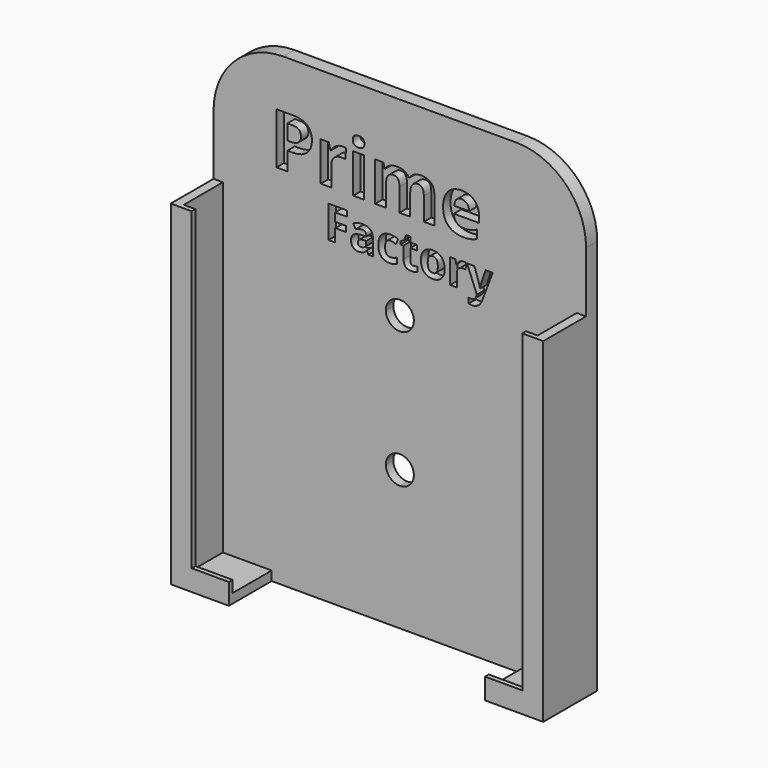
from build123d import *

# Parameters (mm, degrees)
F1_DEPTH        = 13
F3_DEPTH        = 3
F4_W            = 71
F4_H            = 4.5
F5_DEPTH        = 1
F6_R            = 15
F7_W            = 15
F7_H            = 4.5
F8_DEPTH        = 11
F10_W           = 24
F10_H           = 43
F11_DEPTH       = 1
F13_DEPTH       = 0.5
F14_DEPTH       = 30
F15_DEPTH       = 26
F16_DEPTH       = 8
F17_DEPTH       = 8
F18_TEXT_SIZE   = 15.3918698844
F18_TEXT_SIZE_2 = 9.6479482535
F19_DEPTH       = 2
F20_DEPTH       = 0.5
F21_DEPTH       = 0.5
F22_DEPTH       = 0.5
F23_DEPTH       = 0.5
F27_DEPTH       = 25
F28_DEPTH       = 25


# Not quite as in the source:
# - Text() gives the source's letters only with a copy of the font that has no kerning and outlines rounded to 1/6400 em; it was checked with that copy


with BuildPart() as f1:
    # F0 (on Front) → F1 (new body)
    with BuildSketch(Plane.XZ):
        Polygon((-38, -35), (-38, 35), (-40, 35), (-40, -37), (40, -37), (40, 35), (38, 35), (38, -35), align=None)
    extrude(amount=F1_DEPTH)

    # F2 (on face) → F3 (join)
    with BuildSketch(Plane(origin=(0, 0, 0), x_dir=(-1, 0, 0), z_dir=(0, 1, 0))):
        Polygon((-40, 63), (-40, 35), (-38, 35), (-38, -35), (38, -35), (38, 35), (40, 35), (40, 63), align=None)
    extrude(amount=-F3_DEPTH)

    # F4 (on face) → F5 (join)
    with BuildSketch(Plane.XZ.offset(13)):
        Polygon((35.5, -37), (40, -37), (40, 35), (35.5, 35), (35.5, -32.5), align=None)
        with Locations((0, -34.75)):
            Rectangle(F4_W, F4_H)
        Polygon((-40, -37), (-35.5, -37), (-35.5, -32.5), (-35.5, 35), (-40, 35), align=None)
    extrude(amount=F5_DEPTH)

    # F6
    f6_edges = [f1.edges().sort_by_distance(p)[0] for p in [
        (-40, -1.5, 63),
        (40, -1.5, 63),
    ]]
    fillet(f6_edges, radius=F6_R)

    # F7 (on face) → F8 (cut)
    with BuildSketch(Plane.XZ.offset(14)):
        with Locations((1.9808986038, -34.75)):
            Rectangle(F7_W, F7_H)
    extrude(amount=-F8_DEPTH, mode=Mode.SUBTRACT)

    # F10 (on face) → F11 (cut)
    with BuildSketch(Plane(origin=(0, 0, 0), x_dir=(-1, 0, 0), z_dir=(0, 1, 0))):
        with Locations((0, 7.5584797218)):
            Rectangle(F10_W, F10_H)
    extrude(amount=-F11_DEPTH, mode=Mode.SUBTRACT)

    # F12 (on face) → F13 (cut)
    with BuildSketch(Plane.XZ.offset(3)):
        with BuildLine():
            Line((-38, 35), (-38, -35))
            Line((-38, -35), (-5.5191013962, -35))
            Line((-5.5191013962, -35), (9.4808986038, -35))
            Line((9.4808986038, -35), (38, -35))
            Line((38, -35), (38, 35))
            Line((38, 35), (40, 35))
            Line((40, 35), (40, 48))
            ThreePointArc((40, 48), (35.6066017178, 58.6066017178), (25, 63))
            Line((25, 63), (-25, 63))
            ThreePointArc((-25, 63), (-35.6066017178, 58.6066017178), (-40, 48))
            Line((-40, 48), (-40, 35))
            Line((-40, 35), (-38, 35))
        make_face()
    extrude(amount=F13_DEPTH, mode=Mode.SUBTRACT)

    # F14 (cut): a face of the model
    f14_faces = [f1.faces().sort_by_distance(p)[0] for p in [
        (-5.5191013962, -9.0102040816, -35.7704081633),
    ]]
    extrude(f14_faces, amount=-F14_DEPTH, mode=Mode.SUBTRACT)

    # F15 (cut): a face of the model
    f15_faces = [f1.faces().sort_by_distance(p)[0] for p in [
        (9.4808986038, -9.0102040816, -35.7704081633),
    ]]
    extrude(f15_faces, amount=-F15_DEPTH, mode=Mode.SUBTRACT)

    # F16 (add): a face of the model
    f16_faces = [f1.faces().sort_by_distance(p)[0] for p in [
        (35.4808986038, -9.0102040816, -35.7704081633),
    ]]
    extrude(f16_faces, amount=F16_DEPTH)

    # F17 (add): a face of the model
    f17_faces = [f1.faces().sort_by_distance(p)[0] for p in [
        (-35.5191013962, -9.0102040816, -35.7704081633),
    ]]
    extrude(f17_faces, amount=F17_DEPTH)

    # F18 (on face) → F19 (cut)
    with BuildSketch(Plane.XZ.offset(3)):
        with Locations((-27.8627396328, 41.5634587407)):
            Text('Prime', F18_TEXT_SIZE, font='Open Sans', font_style=FontStyle.BOLD, text_align=(TextAlign.LEFT, TextAlign.BOTTOM))
        with Locations((-16.1838065833, 31.4543135464)):
            Text('Factory', F18_TEXT_SIZE_2, font='Open Sans', font_style=FontStyle.BOLD, text_align=(TextAlign.LEFT, TextAlign.BOTTOM))
    extrude(amount=-F19_DEPTH, mode=Mode.SUBTRACT)

    # F20 (cut): a face of the model
    f20_faces = [f1.faces().sort_by_distance(p)[0] for p in [
        (12, -0.5, 7.5584797218),
    ]]
    extrude(f20_faces, amount=-F20_DEPTH, mode=Mode.SUBTRACT)

    # F21 (cut): a face of the model
    f21_faces = [f1.faces().sort_by_distance(p)[0] for p in [
        (-12, -0.5, 7.5584797218),
    ]]
    extrude(f21_faces, amount=-F21_DEPTH, mode=Mode.SUBTRACT)

    # F22 (add): faces of the model
    f22_faces = [f1.faces().sort_by_distance(p)[0] for p in [
        (-37.1272964046, -14, -4.3677457065),
        (37.122700132, -14, -4.3822508301),
    ]]
    extrude(f22_faces, amount=F22_DEPTH)

    # F23 (cut): faces of the model
    f23_faces = [f1.faces().sort_by_distance(p)[0] for p in [
        (-36.2136700107, -13, -3.4541193126),
        (36.2094032796, -13, -3.4689539777),
    ]]
    extrude(f23_faces, amount=-F23_DEPTH, mode=Mode.SUBTRACT)

    # F26 (on face) → F27 (cut)
    with BuildSketch(Plane(origin=(0, -1, 0), x_dir=(-1, 0, 0), z_dir=(0, 1, 0))):
        with BuildLine():
            ThreePointArc((0, 25.1642662283), (-2.1243704896, 20.0355821807), (3.0043135579, 22.1599526703))
            ThreePointArc((3.0043135579, 22.1599526703), (2.1243704896, 24.28432316), (0, 25.1642662283))
        make_face()
        with BuildLine():
            ThreePointArc((0, -10.0390259604), (2.1259519358, -9.1584278357), (3.0065500605, -7.0324758999))
            ThreePointArc((3.0065500605, -7.0324758999), (-2.1259519358, -4.9065239641), (0, -10.0390259604))
        make_face()
    extrude(amount=-F27_DEPTH, mode=Mode.SUBTRACT)

    # F26 (on face) → F28 (cut)
    with BuildSketch(Plane(origin=(0, -1, 0), x_dir=(-1, 0, 0), z_dir=(0, 1, 0))):
        with BuildLine():
            ThreePointArc((0, 25.1642662283), (-2.1243704896, 20.0355821807), (3.0043135579, 22.1599526703))
            ThreePointArc((3.0043135579, 22.1599526703), (2.1243704896, 24.28432316), (0, 25.1642662283))
        make_face()
        with BuildLine():
            ThreePointArc((0, -10.0390259604), (2.1259519358, -9.1584278357), (3.0065500605, -7.0324758999))
            ThreePointArc((3.0065500605, -7.0324758999), (-2.1259519358, -4.9065239641), (0, -10.0390259604))
        make_face()
    extrude(amount=-F28_DEPTH, mode=Mode.SUBTRACT)


solid = f1.part
